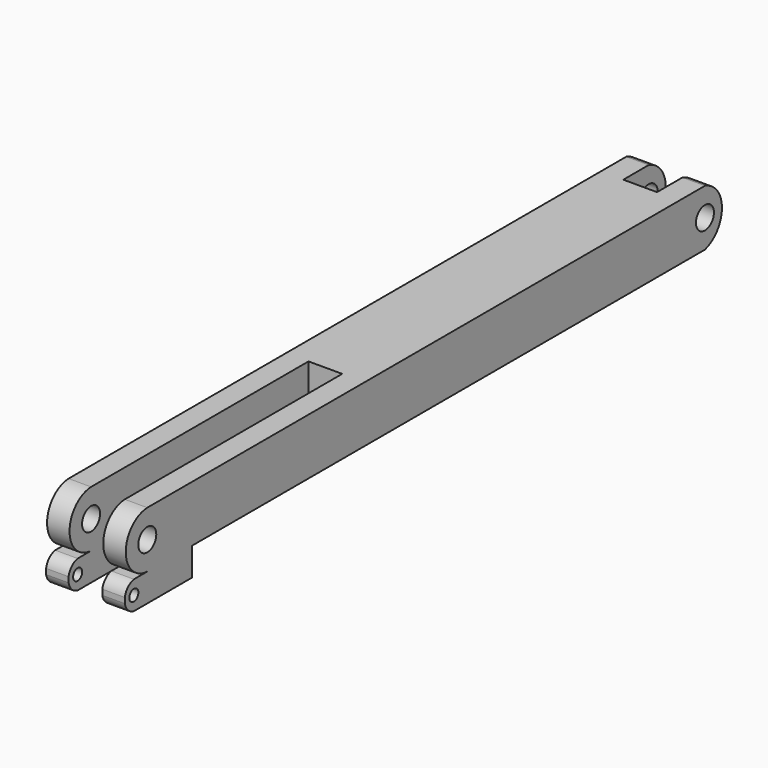
from build123d import *

# Parameters (mm, degrees)
F0_W      = 63.5
F0_H      = 12.7
F1_DEPTH  = 17.78
F2_W      = 5.08
F2_H      = 12.7
F3_DEPTH  = 25.4
F4_R      = 2.54
F5_DEPTH  = 25.4
F6_DEPTH  = 50.8
F7_DEPTH  = 76.2
F8_W      = 5.08
F8_H      = 12.7
F9_DEPTH  = 12.7
F11_W     = 5.08
F11_H     = 12.7
F12_DEPTH = 6.35
F13_DEPTH = 6.35
F15_DEPTH = 25.4
F10_R     = 2.54
F16_DEPTH = 25.4
F14_R     = 1.2823476499
F17_DEPTH = 25.4


# Not quite as in the source:
# - a feature names something its author has since deleted; it is built from what else it names


with BuildPart() as f1:
    # F0 (on Right) → F1 (new body)
    with BuildSketch(Plane.YZ):
        with Locations((10.0746992975, -1.9877629941)):
            Rectangle(F0_W, F0_H)
    extrude(amount=F1_DEPTH)

    # F2 (on face) → F3 (join)
    with BuildSketch(Plane.XZ.offset(21.6753007025)):
        with Locations((2.54, -1.9877629941)):
            Rectangle(F2_W, F2_H)
        with Locations((15.24, -1.9877629941)):
            Rectangle(F2_W, F2_H)
    extrude(amount=F3_DEPTH)

    # F4 (on face) → F5 (cut)
    with BuildSketch(Plane.YZ.offset(17.78)):
        with Locations((-32.2765819728, -1.9877629941)):
            Circle(F4_R)
        with BuildLine():
            ThreePointArc((-32.2765819728, -8.3377629941), (-38.3512132445, -1.9877629941), (-32.2765819728, 4.3622370059))
            Line((-32.2765819728, 4.3622370059), (-47.0753007025, 4.3622370059))
            Line((-47.0753007025, 4.3622370059), (-47.0753007025, -8.3377629941))
            Line((-47.0753007025, -8.3377629941), (-32.2765819728, -8.3377629941))
        make_face()
    extrude(amount=-F5_DEPTH, mode=Mode.SUBTRACT)

    # F6 (cut): a face of the model
    f6_faces = [f1.faces().sort_by_distance(p)[0] for p in [
        (8.89, -21.6753007025, -1.9877629941),
    ]]
    extrude(f6_faces, amount=-F6_DEPTH, mode=Mode.SUBTRACT)

    # F7 (add): a face of the model
    f7_faces = [f1.faces().sort_by_distance(p)[0] for p in [
        (8.89, 41.8246992975, -1.9877629941),
    ]]
    extrude(f7_faces, amount=F7_DEPTH)

    # F8 (on face) → F9 (join)
    with BuildSketch(Plane(origin=(0, 118.0246992975, 0), x_dir=(-1, 0, 0), z_dir=(0, 1, 0))):
        with Locations((-15.24, -1.9877629941)):
            Rectangle(F8_W, F8_H)
        with Locations((-2.54, -1.9877629941)):
            Rectangle(F8_W, F8_H)
    extrude(amount=F9_DEPTH)

    # F11 (on face) → F12 (join)
    with BuildSketch(Plane(origin=(0, 0, -8.3377629941), x_dir=(1, 0, 0), z_dir=(0, 0, -1))):
        with Locations((15.24, 25.9265819728)):
            Rectangle(F11_W, F11_H)
        with Locations((2.54, 25.9265819728)):
            Rectangle(F11_W, F11_H)
    extrude(amount=F12_DEPTH)

    # F13 (add): faces of the model
    f13_faces = [f1.faces().sort_by_distance(p)[0] for p in [
        (15.24, -32.2765819728, -11.5127629941),
        (2.54, -32.2765819728, -11.5127629941),
    ]]
    extrude(f13_faces, amount=F13_DEPTH)

    # F14 (on face) → F15 (cut)
    with BuildSketch(Plane.YZ.offset(17.78)):
        with BuildLine():
            ThreePointArc((-38.6265819728, -10.9001689166), (-37.7400292742, -9.2277758835), (-36.0694751143, -8.3377629941))
            Line((-36.0694751143, -8.3377629941), (-38.6265819728, -8.3377629941))
            Line((-38.6265819728, -8.3377629941), (-38.6265819728, -10.9001689166))
        make_face()
        with BuildLine():
            ThreePointArc((-36.0694751143, -14.6877629941), (-37.7400292742, -13.7977501047), (-38.6265819728, -12.1253570717))
            Line((-38.6265819728, -12.1253570717), (-38.6265819728, -14.6877629941))
            Line((-38.6265819728, -14.6877629941), (-36.0694751143, -14.6877629941))
        make_face()
    extrude(amount=-F15_DEPTH, mode=Mode.SUBTRACT)

    # F10 (on face) → F16 (cut)
    with BuildSketch(Plane.YZ.offset(17.78)):
        with BuildLine():
            ThreePointArc((125.2040266991, 4.3622370059), (130.0066745518, -1.9877629941), (125.2040266991, -8.3377629941))
            Line((125.2040266991, -8.3377629941), (130.7246992975, -8.3377629941))
            Line((130.7246992975, -8.3377629941), (130.7246992975, 4.3622370059))
            Line((130.7246992975, 4.3622370059), (125.2040266991, 4.3622370059))
        make_face()
        with Locations((125.2040266991, -1.9877629941)):
            Circle(F10_R)
    extrude(amount=-F16_DEPTH, mode=Mode.SUBTRACT)

    # F14 (on face) → F17 (cut)
    with BuildSketch(Plane.YZ.offset(17.78)):
        with Locations((-36.0694751144, -11.5127629941)):
            Circle(F14_R)
    extrude(amount=-F17_DEPTH, mode=Mode.SUBTRACT)


solid = f1.part
